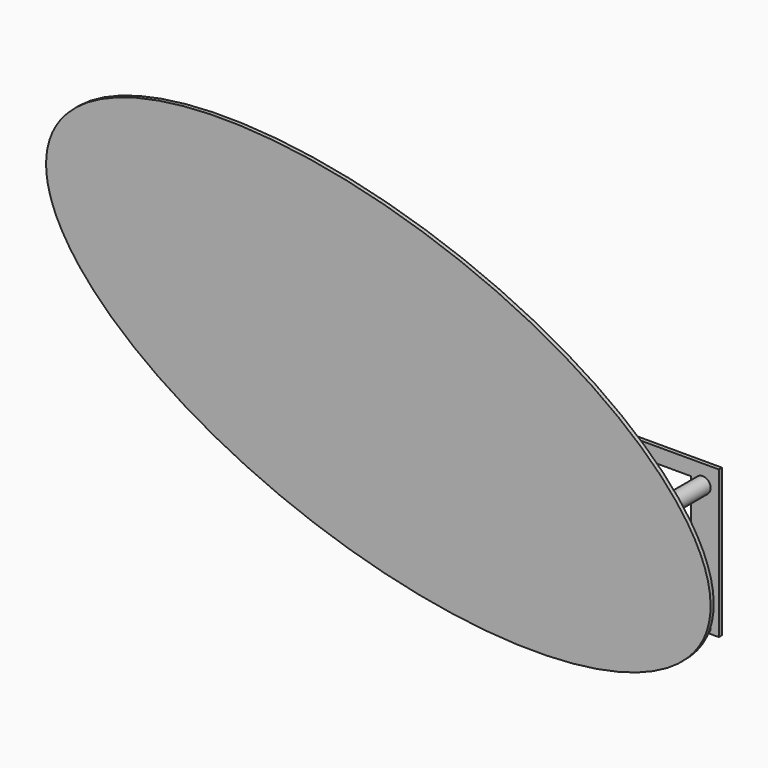
from build123d import *

# Parameters (mm, degrees)
F0_W     = 130.637280643
F0_H     = 74.935246259
F0_W_2   = 105.6843772531
F0_H_2   = 55.9340212494
F1_DEPTH = 2
F2_R     = 4.0448903619
F3_DEPTH = 25
F5_DEPTH = 2


# Not quite as in the source:
# - a pattern or mirror of a feature is missing from the dataset's text; its kind, count and spacing are read off the source's solid


with BuildPart() as f1:
    # F0 (on Front) → F1 (new body)
    with BuildSketch(Plane.XZ):
        with Locations((1.5145130455, 3.4574959427)):
            Rectangle(F0_W, F0_H)
        with Locations((0, 5.3404411301)):
            Rectangle(F0_W_2, F0_H_2, mode=Mode.SUBTRACT)
    extrude(amount=F1_DEPTH)

    # F2 (on face) → F3 (join)
    with BuildSketch(Plane.XZ.offset(2)):
        with Locations((-58.6657784879, 31.2389582396)):
            Circle(F2_R)
    f3 = extrude(amount=F3_DEPTH)

    # F3_copies: F3 across plane
    add(f3.mirror(Plane(origin=(0, 0, 0), x_dir=(0, 0, 1), z_dir=(1, 0, 0))))

    # F3_copies1: F3 across plane
    add(f3.mirror(Plane(origin=(0, 0, 0), x_dir=(-1, 0, 0), z_dir=(0, 0, -1))))

    # F3_copies2: F3 across plane
    add(f3.mirror(Plane(origin=(0, 0, 0), x_dir=(0.4700088099, 0, 0.8826617238), z_dir=(0.8826617238, 0, -0.4700088099))))


with BuildPart() as f5:
    # F4 (on face) → F5 (new body)
    with BuildSketch(Plane.XZ.offset(27)):
        with BuildLine():
            add(Edge.make_bspline(
                [(82.4152380228, -15.0861563161), (125.6547061385, 114.6322429601), (-146.1206258445, 133.15824589), (-417.8959578276, 151.6842488199), (-189.3600939602, 3.4398466138), (39.1757699071, -144.8045555923), (82.4152380228, -15.0861563161)],
                knots=[0, 0, 0, 2.0943951024, 2.0943951024, 4.1887902048, 4.1887902048, 6.2831853072, 6.2831853072, 6.2831853072], degree=2, weights=[1, 0.5, 1, 0.5, 1, 0.5, 1]))
        make_face()
    extrude(amount=F5_DEPTH)


solid = Compound([f1.part, f5.part])
